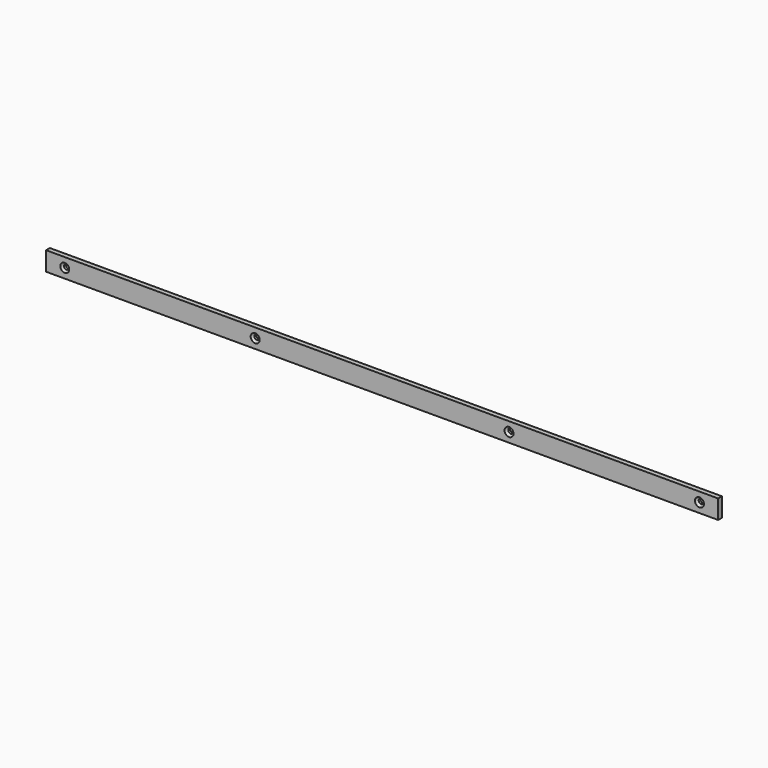
from build123d import *

# Parameters (mm, degrees)
F0_W     = 900
F0_H     = 25.4
F0_R     = 3.25
F1_DEPTH = 6.35
F2_SIZE  = 2.75
F3_SIZE  = 0.5


with BuildPart() as f1:
    # F0 (on Front) → F1 (new body)
    with BuildSketch(Plane.XZ):
        Rectangle(F0_W, F0_H)
        with Locations((-425, 0)):
            Circle(F0_R, mode=Mode.SUBTRACT)
        with Locations((-170, 0)):
            Circle(F0_R, mode=Mode.SUBTRACT)
        with Locations((170, 0)):
            Circle(F0_R, mode=Mode.SUBTRACT)
        with Locations((425, 0)):
            Circle(F0_R, mode=Mode.SUBTRACT)
    extrude(amount=F1_DEPTH)

    # F2
    f2_edges = [f1.edges().sort_by_distance(p)[0] for p in [
        (-428.25, -6.35, 0),
        (-173.25, -6.35, 0),
        (166.75, -6.35, 0),
        (421.75, -6.35, 0),
    ]]
    chamfer(f2_edges, length=F2_SIZE)

    # F3
    f3_edges = [f1.edges().sort_by_distance(p)[0] for p in [
        (421.75, 0, 0),
        (166.75, 0, 0),
        (-173.25, 0, 0),
        (-428.25, 0, 0),
    ]]
    chamfer(f3_edges, length=F3_SIZE)


solid = f1.part
